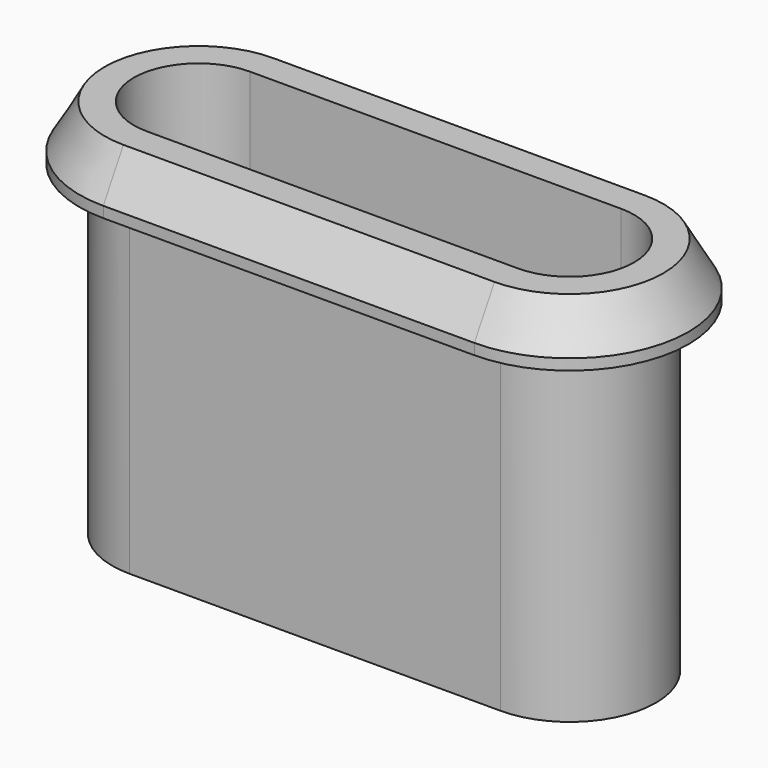
from build123d import *

# Parameters (mm, degrees)
F1_DEPTH    = 30
F3_DEPTH    = 5
F4_T1_DEPTH = 34.125
F4_T4_ANGLE = 180
F4_T6_ANGLE = 180


# Not quite as in the source:
# - a fillet or chamfer that OpenCascade refuses, or shapes differently, is made with other operations: its cross-section is extruded or revolved along the edge and cut away or added


with BuildPart() as f1:
    # F0 (on Top) → F1 (new body)
    with BuildSketch(Plane.XY):
        with BuildLine():
            Line((-17.0625, -7.9375), (0, -7.9375))
            Line((0, -7.9375), (17.0625, -7.9375))
            ThreePointArc((17.0625, -7.9375), (25, 0), (17.0625, 7.9375))
            Line((17.0625, 7.9375), (0, 7.9375))
            Line((0, 7.9375), (-17.0625, 7.9375))
            ThreePointArc((-17.0625, 7.9375), (-25, 0), (-17.0625, -7.9375))
        make_face()
        with BuildLine():
            Line((-17.0625, 5.9375000447), (0, 5.9375000447))
            Line((0, 5.9375000447), (17.0625, 5.9375000447))
            ThreePointArc((17.0625, 5.9375000447), (23.0000000447, 0), (17.0625, -5.9375000447))
            Line((17.0625, -5.9375000447), (0, -5.9375000447))
            Line((0, -5.9375000447), (-17.0625, -5.9375000447))
            ThreePointArc((-17.0625, -5.9375000447), (-23.0000000447, 0), (-17.0625, 5.9375000447))
        make_face(mode=Mode.SUBTRACT)
    extrude(amount=F1_DEPTH)

    # F2 (on face) → F3 (join)
    with BuildSketch(Plane.XY.offset(30)):
        with BuildLine():
            ThreePointArc((17.0625, -10.9375000447), (28.0000000447, 0), (17.0625, 10.9375000447))
            Line((17.0625, 10.9375000447), (-17.0625, 10.9375000447))
            ThreePointArc((-17.0625, 10.9375000447), (-28.0000000447, 0), (-17.0625, -10.9375000447))
            Line((-17.0625, -10.9375000447), (17.0625, -10.9375000447))
        make_face()
        with BuildLine():
            Line((17.0625, -7.9375), (-17.0625, -7.9375))
            ThreePointArc((-17.0625, -7.9375), (-25, 0), (-17.0625, 7.9375))
            Line((-17.0625, 7.9375), (17.0625, 7.9375))
            ThreePointArc((17.0625, 7.9375), (25, 0), (17.0625, -7.9375))
        make_face(mode=Mode.SUBTRACT)
        with BuildLine():
            ThreePointArc((-17.0625, 7.9375), (-25, 0), (-17.0625, -7.9375))
            Line((-17.0625, -7.9375), (17.0625, -7.9375))
            ThreePointArc((17.0625, -7.9375), (25, 0), (17.0625, 7.9375))
            Line((17.0625, 7.9375), (-17.0625, 7.9375))
        make_face()
        with BuildLine():
            Line((-17.0625, 5.9375000447), (17.0625, 5.9375000447))
            ThreePointArc((17.0625, 5.9375000447), (23.0000000447, 0), (17.0625, -5.9375000447))
            Line((17.0625, -5.9375000447), (-17.0625, -5.9375000447))
            ThreePointArc((-17.0625, -5.9375000447), (-23.0000000447, 0), (-17.0625, 5.9375000447))
        make_face(mode=Mode.SUBTRACT)
    extrude(amount=F3_DEPTH)

    # F4: chamfer of 4 x 2.3094010768 on 4 edges, made by hand

    # F4_s2 → F4_t1 (cut)
    with BuildSketch(Plane.YZ.offset(-17.0625)):
        Polygon((-8.6280989679, 35), (-10.9375000447, 31), (-10.9375000447, 35), align=None)
        Polygon((8.6280989679, 35), (10.9375000447, 31), (10.9375000447, 35), align=None)
    extrude(amount=F4_T1_DEPTH, mode=Mode.SUBTRACT)

    # F4_s3 → F4_t4 (revolve, cut)
    with BuildSketch(Plane.YZ.offset(-17.0625)):
        Polygon((8.6280989679, 35), (10.9375000447, 31), (10.9375000447, 35), align=None)
    revolve(axis=Axis((-17.0625, 0, 35), (0, 0, 1)), revolution_arc=F4_T4_ANGLE, mode=Mode.SUBTRACT)

    # F4_s5 → F4_t6 (revolve, cut)
    with BuildSketch(Plane.YZ.offset(17.0625)):
        Polygon((-8.6280989679, 35), (-10.9375000447, 31), (-10.9375000447, 35), align=None)
    revolve(axis=Axis((17.0625, 0, 35), (0, 0, 1)), revolution_arc=F4_T6_ANGLE, mode=Mode.SUBTRACT)


solid = f1.part
